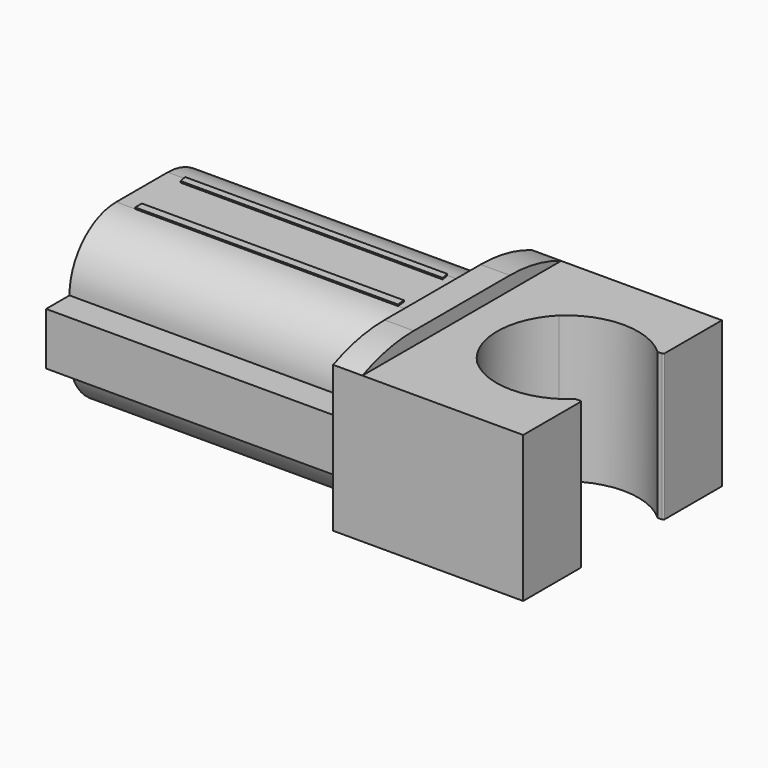
from build123d import *

# Parameters (mm, degrees)
F1_DEPTH    = 1.27
F2_R        = 0.0254
F4_DEPTH    = 0.508
F5_T1_DEPTH = 5.1142141328
F5_T3_DEPTH = 4.5716483018
F5_T5_DEPTH = 5.8519702279
F5_T7_DEPTH = 5.3913281872
F6_W        = 3.1516760678
F6_H        = 2.9446112536
F7_DEPTH    = 5.08
F8_T1_DEPTH = 7.62
F10_DEPTH   = 0.0254
F11_W       = 4.6949440148
F11_H       = 0.1139125334
F12_DEPTH   = 0.0254
F13_W       = 5.08
F13_H       = 0.9126112536
F14_DEPTH   = 0.508
F15_W       = 5.08
F15_H       = 0.9126112536
F16_DEPTH   = 0.508


# Not quite as in the source:
# - a fillet or chamfer that OpenCascade refuses, or shapes differently, is made with other operations: its cross-section is extruded or revolved along the edge and cut away or added


with BuildPart() as f1:
    # F0 (on Top) → F1 (new body, symmetric)
    with BuildSketch(Plane.XY):
        with BuildLine():
            Line((0.914706802, 2.159), (-1.879293198, 2.159))
            Line((-1.879293198, 2.159), (-1.879293198, -2.159))
            Line((-1.879293198, -2.159), (0.914706802, -2.159))
            Line((0.914706802, -2.159), (0.914706802, -0.889))
            Line((0.914706802, -0.889), (0.863906802, -0.889))
            Line((0.863906802, -0.889), (0.813106802, -0.889))
            ThreePointArc((0.813106802, -0.889), (-0.0443418563, -1.2221163224), (-0.901769336, -0.8889454908))
            ThreePointArc((-0.901769336, -0.8889454908), (-1.2648079256, 5.45092e-05), (-0.901769336, 0.8890545092))
            ThreePointArc((-0.901769336, 0.8890545092), (-0.0443206777, 1.2221708316), (0.813106802, 0.889))
            Line((0.813106802, 0.889), (0.863906802, 0.889))
            Line((0.863906802, 0.889), (0.914706802, 0.889))
            Line((0.914706802, 0.889), (0.914706802, 2.159))
        make_face()
    extrude(amount=F1_DEPTH, both=True)

    # F2
    f2_edges = [f1.edges().sort_by_distance(p)[0] for p in [
        (0.914707, 0.889, 0),
        (0.914707, -0.889, 0),
    ]]
    fillet(f2_edges, radius=F2_R)

    # F3 (on face) → F4 (join)
    with BuildSketch(Plane(origin=(-1.879293198, 0, 0), x_dir=(0, -1, 0), z_dir=(-1, 0, 0))):
        Polygon((-1.9648331217, 1.5023018932), (-2.159, 1.27), (-2.159, -1.27), (-1.9496894674, -1.5794709325), (1.8575610593, -1.5794709325), (2.159, -1.27), (2.159, 1.27), (1.8563199556, 1.5023018932), align=None)
    extrude(amount=F4_DEPTH)

    # F5: fillet of radius 2.794 on 4 edges, made by hand

    # F5_s2 → F5_t1 (cut)
    with BuildSketch(Plane.YZ.offset(-4.6904002644)):
        with BuildLine():
            ThreePointArc((1.0435902952, 1.5023018932), (1.6132619065, 1.4436099664), (2.159, 1.27))
            Line((2.159, 1.27), (1.9648331217, 1.5023018932))
            Line((1.9648331217, 1.5023018932), (1.0435902952, 1.5023018932))
        make_face()
    extrude(amount=F5_T1_DEPTH, mode=Mode.SUBTRACT)

    # F5_s4 → F5_t3 (cut)
    with BuildSketch(Plane.YZ.offset(-4.4191173489)):
        with BuildLine():
            ThreePointArc((-1.0435902952, 1.5023018932), (-1.6132619065, 1.4436099664), (-2.159, 1.27))
            Line((-2.159, 1.27), (-1.8563199556, 1.5023018932))
            Line((-1.8563199556, 1.5023018932), (-1.0435902952, 1.5023018932))
        make_face()
    extrude(amount=F5_T3_DEPTH, mode=Mode.SUBTRACT)

    # F5_s6 → F5_t5 (cut)
    with BuildSketch(Plane.YZ.offset(-5.0592783119)):
        with BuildLine():
            ThreePointArc((0.8808954219, -1.5794709325), (1.5384141613, -1.5010012872), (2.159, -1.27))
            Line((2.159, -1.27), (1.9496894674, -1.5794709325))
            Line((1.9496894674, -1.5794709325), (0.8808954219, -1.5794709325))
        make_face()
    extrude(amount=F5_T5_DEPTH, mode=Mode.SUBTRACT)

    # F5_s8 → F5_t7 (cut)
    with BuildSketch(Plane.YZ.offset(-4.8289572916)):
        with BuildLine():
            ThreePointArc((-2.159, -1.27), (-1.5384141613, -1.5010012872), (-0.8808954219, -1.5794709325))
            Line((-0.8808954219, -1.5794709325), (-1.8575610593, -1.5794709325))
            Line((-1.8575610593, -1.5794709325), (-2.159, -1.27))
        make_face()
    extrude(amount=F5_T7_DEPTH, mode=Mode.SUBTRACT)

    # F6 (on face) → F7 (join)
    with BuildSketch(Plane(origin=(-2.387293198, 0, 0), x_dir=(0, -1, 0), z_dir=(-1, 0, 0))):
        with Locations((-0.0374238726, -0.0286956604)):
            Rectangle(F6_W, F6_H)
    extrude(amount=F7_DEPTH)

    # F8: fillet of radius 1.016 on 4 edges, made by hand

    # F8_s2 → F8_t1 (cut)
    with BuildSketch(Plane.YZ.offset(-10.007293198)):
        with BuildLine():
            ThreePointArc((1.6132619065, 0.4276099664), (1.3156823962, 1.1460304561), (0.5972619065, 1.4436099664))
            Line((0.5972619065, 1.4436099664), (1.6132619065, 1.4436099664))
            Line((1.6132619065, 1.4436099664), (1.6132619065, 0.4276099664))
        make_face()
        with BuildLine():
            ThreePointArc((-1.5384141613, 0.4276099664), (-1.240834651, 1.1460304561), (-0.5224141613, 1.4436099664))
            Line((-0.5224141613, 1.4436099664), (-1.5384141613, 1.4436099664))
            Line((-1.5384141613, 1.4436099664), (-1.5384141613, 0.4276099664))
        make_face()
        with BuildLine():
            ThreePointArc((1.6132619065, -0.4850012872), (1.3156823962, -1.2034217769), (0.5972619065, -1.5010012872))
            Line((0.5972619065, -1.5010012872), (1.6132619065, -1.5010012872))
            Line((1.6132619065, -1.5010012872), (1.6132619065, -0.4850012872))
        make_face()
        with BuildLine():
            ThreePointArc((-1.5384141613, -0.4850012872), (-1.240834651, -1.2034217769), (-0.5224141613, -1.5010012872))
            Line((-0.5224141613, -1.5010012872), (-1.5384141613, -1.5010012872))
            Line((-1.5384141613, -1.5010012872), (-1.5384141613, -0.4850012872))
        make_face()
    extrude(amount=F8_T1_DEPTH, mode=Mode.SUBTRACT)

    # F9 (on face) → F10 (join)
    with BuildSketch(Plane.XY.offset(1.4436099664)):
        Polygon((-7.1662743576, 0.5972619065), (-7.1378163993, 0.466715981), (-2.5845263153, 0.466715981), (-2.609875286, 0.5972619065), align=None)
        Polygon((-2.5695776567, -0.5224141613), (-2.5845263153, -0.3768240858), (-7.1378163993, -0.3768240858), (-7.1378163993, -0.5224141613), align=None)
    extrude(amount=F10_DEPTH)

    # F11 (on face) → F12 (join)
    with BuildSketch(Plane(origin=(0, 0, -1.5010012872), x_dir=(1, 0, 0), z_dir=(0, 0, -1))):
        Polygon((-7.2172759101, 0.376087494), (-2.5223318953, 0.4174394126), (-2.5223318953, 0.5224141613), (-7.2172759101, 0.5224141613), align=None)
        with Locations((-4.8698039027, -0.5403056398)):
            Rectangle(F11_W, F11_H)
    extrude(amount=F12_DEPTH)

    # F13 (on face) → F14 (join)
    with BuildSketch(Plane(origin=(0, 1.6132619065, 0), x_dir=(-1, 0, 0), z_dir=(0, 1, 0))):
        with Locations((4.927293198, -0.0286956604)):
            Rectangle(F13_W, F13_H)
    extrude(amount=F14_DEPTH)

    # F15 (on face) → F16 (join)
    with BuildSketch(Plane.XZ.offset(1.5384141613)):
        with Locations((-4.927293198, -0.0286956604)):
            Rectangle(F15_W, F15_H)
    extrude(amount=F16_DEPTH)


solid = f1.part
